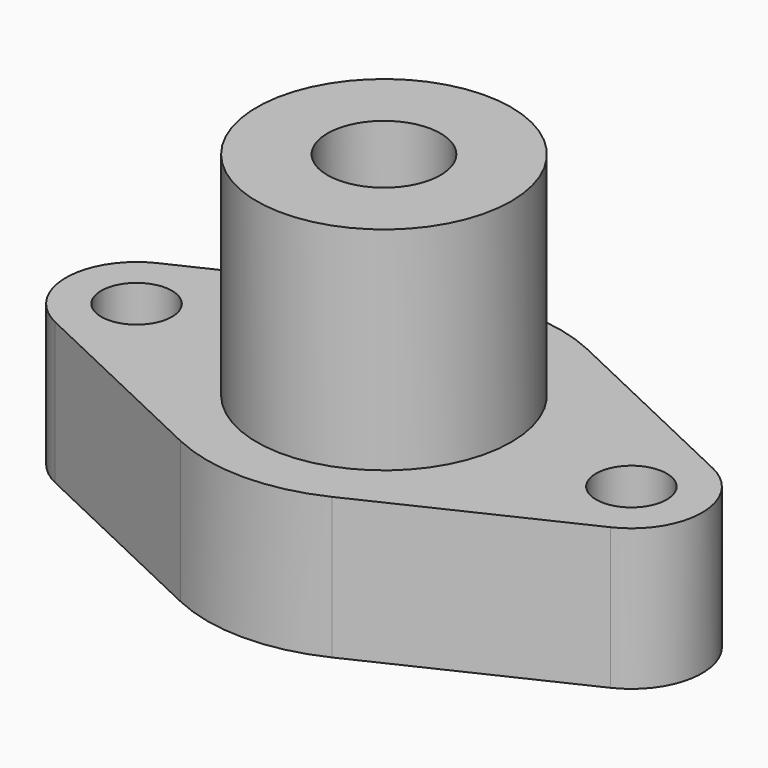
from build123d import *

# Parameters (mm, degrees)
F1_DEPTH       = 20
F2_R           = 18
F3_DEPTH       = 30
F5_D           = 10
F5_DEPTH       = 20
F5_TIP         = 3.0043030951
F5_ON_F4_D     = 10
F5_ON_F4_DEPTH = 20
F5_ON_F4_TIP   = 3.0043030951
F7_D           = 16
F7_DEPTH       = 25
F7_TIP         = 4.8068849522
F8_T1_DEPTH    = 79.2927061282
F9_R           = 10


# Not quite as in the source:
# - a fillet or chamfer that OpenCascade refuses, or shapes differently, is made with other operations: its cross-section is extruded or revolved along the edge and cut away or added


with BuildPart() as f1:
    # F0 (on Top) → F1 (new body)
    with BuildSketch(Plane.XY):
        with BuildLine():
            Line((-25, 0), (0, 0))
            Line((0, 0), (25, 0))
            ThreePointArc((25, 0), (21.1288562998, 13.3630622038), (10.7142854831, 22.5876976823))
            ThreePointArc((10.7142854831, 22.5876976823), (-9.67e-08, 25), (-10.7142856578, 22.5876975994))
            ThreePointArc((-10.7142856578, 22.5876975994), (-21.1288563515, 13.363062122), (-25, 0))
        make_face()
        with BuildLine():
            Line((25, 0), (0, 0))
            Line((0, 0), (-25, 0))
            ThreePointArc((-25, 0), (-21.128856388, -13.3630620643), (-10.7142857812, -22.5876975409))
            ThreePointArc((-10.7142857812, -22.5876975409), (-4.6e-08, -25), (10.7142856981, -22.5876975803))
            ThreePointArc((10.7142856981, -22.5876975803), (21.1288563634, -13.3630621032), (25, 0))
        make_face()
        with BuildLine():
            ThreePointArc((10.7142854831, 22.5876976823), (21.1288562998, 13.3630622038), (25, 0))
            ThreePointArc((25, 0), (29.6547751302, 8.4515425273), (39.2857142182, 9.0350790611))
            Line((39.2857142182, 9.0350790611), (10.7142854831, 22.5876976823))
        make_face()
        with BuildLine():
            ThreePointArc((39.2857142182, 9.0350790611), (29.6547751302, 8.4515425273), (25, 0))
            ThreePointArc((25, 0), (29.6547751142, -8.4515425172), (39.285714184, -9.0350790773))
            ThreePointArc((39.285714184, -9.0350790773), (43.4515425172, -5.3452248858), (45, 0))
            ThreePointArc((45, 0), (43.4515425273, 5.3452248698), (39.2857142182, 9.0350790611))
        make_face()
        with BuildLine():
            ThreePointArc((39.285714184, -9.0350790773), (29.6547751142, -8.4515425172), (25, 0))
            ThreePointArc((25, 0), (21.1288563634, -13.3630621032), (10.7142856981, -22.5876975803))
            Line((10.7142856981, -22.5876975803), (39.285714184, -9.0350790773))
        make_face()
        with BuildLine():
            ThreePointArc((-39.2857142392, -9.0350790511), (-29.65477514, -8.4515425335), (-25, 0))
            ThreePointArc((-25, 0), (-29.6547751302, 8.4515425273), (-39.2857142182, 9.0350790611))
            ThreePointArc((-39.2857142182, 9.0350790611), (-45, 1.16e-08), (-39.2857142392, -9.0350790511))
        make_face()
        with BuildLine():
            ThreePointArc((-10.7142857812, -22.5876975409), (-21.128856388, -13.3630620643), (-25, 0))
            ThreePointArc((-25, 0), (-29.65477514, -8.4515425335), (-39.2857142392, -9.0350790511))
            Line((-39.2857142392, -9.0350790511), (-10.7142857812, -22.5876975409))
        make_face()
        with BuildLine():
            ThreePointArc((-39.2857142182, 9.0350790611), (-29.6547751302, 8.4515425273), (-25, 0))
            ThreePointArc((-25, 0), (-21.1288563515, 13.363062122), (-10.7142856578, 22.5876975994))
            Line((-10.7142856578, 22.5876975994), (-39.2857142182, 9.0350790611))
        make_face()
        with BuildLine():
            Line((58.3333333333, 0), (39.2857142182, 9.0350790611))
            ThreePointArc((39.2857142182, 9.0350790611), (43.4515425273, 5.3452248698), (45, 0))
            ThreePointArc((45, 0), (43.4515425172, -5.3452248858), (39.285714184, -9.0350790773))
            Line((39.285714184, -9.0350790773), (58.3333333333, 0))
        make_face()
        with BuildLine():
            ThreePointArc((-10.7142856578, 22.5876975994), (-9.67e-08, 25), (10.7142854831, 22.5876976823))
            Line((10.7142854831, 22.5876976823), (0, 27.6699295265))
            Line((0, 27.6699295265), (-10.7142856578, 22.5876975994))
        make_face()
        with BuildLine():
            Line((0, -27.6699295265), (10.7142856981, -22.5876975803))
            ThreePointArc((10.7142856981, -22.5876975803), (-4.6e-08, -25), (-10.7142857812, -22.5876975409))
            Line((-10.7142857812, -22.5876975409), (0, -27.6699295265))
        make_face()
        with BuildLine():
            ThreePointArc((-39.2857142392, -9.0350790511), (-45, 1.16e-08), (-39.2857142182, 9.0350790611))
            Line((-39.2857142182, 9.0350790611), (-58.3333333333, 0))
            Line((-58.3333333333, 0), (-39.2857142392, -9.0350790511))
        make_face()
    extrude(amount=F1_DEPTH)

    # F2 (on face) → F3 (join)
    with BuildSketch(Plane.XY.offset(20)):
        Circle(F2_R)
    extrude(amount=F3_DEPTH)

    # F5
    with Locations(Plane(origin=(0, 0, 0), x_dir=(1, 0, 0), z_dir=(0, 0, -1))):
        with Locations((-35, 0)):
            Hole(F5_D / 2, depth=F5_DEPTH)
            with Locations((0, 0, -(F5_DEPTH + F5_TIP / 2))):  # 118° drill point
                Cone(0, F5_D / 2, F5_TIP, mode=Mode.SUBTRACT)

    # F5 on F4
    with Locations(Plane(origin=(0, 0, 0), x_dir=(1, 0, 0), z_dir=(0, 0, -1))):
        with Locations((35, 0)):
            Hole(F5_ON_F4_D / 2, depth=F5_ON_F4_DEPTH)
            with Locations((0, 0, -(F5_ON_F4_DEPTH + F5_ON_F4_TIP / 2))):  # 118° drill point
                Cone(0, F5_ON_F4_D / 2, F5_ON_F4_TIP, mode=Mode.SUBTRACT)

    # F7
    with Locations(Plane.XY.offset(50)):
        with Locations((0, 0)):
            Hole(F7_D / 2, depth=F7_DEPTH)
            with Locations((0, 0, -(F7_DEPTH + F7_TIP / 2))):  # 118° drill point
                Cone(0, F7_D / 2, F7_TIP, mode=Mode.SUBTRACT)

    # F8: fillet of radius 25 on 2 edges, made by hand

    # F8_s2 → F8_t1 (cut)
    with BuildSketch(Plane.XY.offset(-29.6463530641)):
        with BuildLine():
            ThreePointArc((10.7142857143, -22.5876975726), (0, -25), (-10.7142857143, -22.5876975726))
            Line((-10.7142857143, -22.5876975726), (0, -27.6699295265))
            Line((0, -27.6699295265), (10.7142857143, -22.5876975726))
        make_face()
        with BuildLine():
            ThreePointArc((10.7142857143, 22.5876975726), (0, 25), (-10.7142857143, 22.5876975726))
            Line((-10.7142857143, 22.5876975726), (0, 27.6699295265))
            Line((0, 27.6699295265), (10.7142857143, 22.5876975726))
        make_face()
    extrude(amount=F8_T1_DEPTH, mode=Mode.SUBTRACT)

    # F9
    f9_edges = [f1.edges().sort_by_distance(p)[0] for p in [
        (-58.333333, 0, 10),
        (58.333333, 0, 10),
    ]]
    fillet(f9_edges, radius=F9_R)


solid = f1.part
